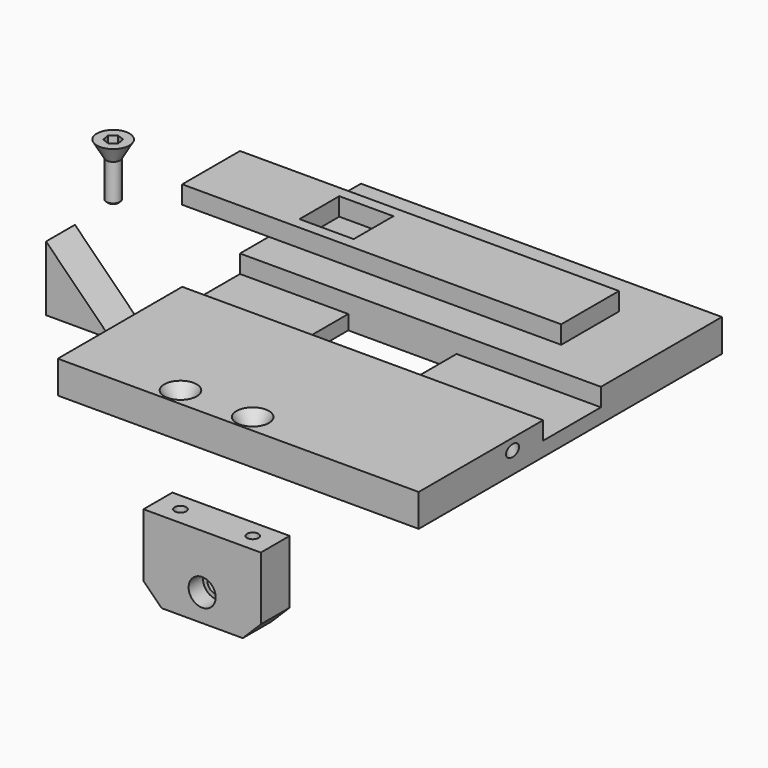
from build123d import *

# Parameters (mm, degrees)
F0_W            = 101.6
F0_H            = 133.35
F1_DEPTH        = 11.43
F3_D            = 4.9149
F3_CSINK_D      = 11.43
F3_CSINK_ANGLE  = 60
F5_W            = 41.275
F5_H            = 12.7
F6_DEPTH        = 28.575
F8_D            = 4.0386
F8_DEPTH        = 9.525
F8_TIP          = 1.213317848
F10_D           = 6.5278
F10_CBORE_D     = 9.525
F10_CBORE_DEPTH = 6.35
F11_W           = 38.1
F11_H           = 25.4
F11_W_2         = 25.4
F12_DEPTH       = 6.35
F13_DEPTH       = 65.406
F15_W           = 101.6
F15_H           = 25.4
F16_DEPTH       = 6.35
F17_W           = 19.05
F17_H           = 17.4752
F18_DEPTH       = 97.156
F20_DEPTH       = 12.7
F21_SIZE2       = 6.34999
F21_SIZE        = 6.34999
F22_DEPTH       = 12.7
F23_DEPTH       = 25.4
F24_DEPTH       = 19.05
F25_SIZE        = 6.35
F28_D           = 4.0386
F28_DEPTH       = 25.4
F28_START       = 31.1992039
F28_TIP         = 1.213317848
F31_SIZE        = 0.508
F33_DEPTH       = 3.175


# Not quite as in the source:
# - a fillet or chamfer is up to 0.001 mm smaller than in the source, because OpenCascade refuses the exact size


with BuildPart() as f1:
    # F0 (on Top) → F1 (new body)
    with BuildSketch(Plane.XY):
        Rectangle(F0_W, F0_H)
    extrude(amount=F1_DEPTH)

    # F3 (through all)
    with Locations(Plane.XY.offset(11.43)):
        with Locations((-12.7, 53.975), (12.7, 53.975), (-12.7, -60.325), (12.7, -60.325)):
            CounterSinkHole(F3_D / 2, F3_CSINK_D / 2, counter_sink_angle=F3_CSINK_ANGLE)

    # F11 (on face) → F12 (cut)
    with BuildSketch(Plane.XY.offset(11.43)):
        with Locations((-31.75, 0.762)):
            Rectangle(F11_W, F11_H)
        with Locations((38.1, 0.762)):
            Rectangle(F11_W_2, F11_H)
    extrude(amount=-F12_DEPTH, mode=Mode.SUBTRACT)

    # F11 (on face) → F13 (cut, through all)
    with BuildSketch(Plane.XY.offset(11.43)):
        with Locations((6.35, 0.762)):
            Rectangle(F11_W, F11_H)
    extrude(amount=-F13_DEPTH, mode=Mode.SUBTRACT)

    # F23 (add): a face of the model
    f23_faces = [f1.faces().sort_by_distance(p)[0] for p in [
        (50.8, 0, 1.338389607),
    ]]
    extrude(f23_faces, amount=F23_DEPTH)

    # F28
    # its depths count from where the whole tool has entered the part; down to there all is cleared
    with Locations(Plane(origin=(71.4375, -71.4375, 0), x_dir=(-0.7071067812, -0.7071067812, 0), z_dir=(0.7071067812, -0.7071067812, 0))):
        with Locations((-35.9150959726, -7.4676)):
            Hole(F28_D / 2, depth=F28_START)
    with Locations(Plane(origin=(71.4375, -71.4375, 0), x_dir=(-0.7071067812, -0.7071067812, 0), z_dir=(0.7071067812, -0.7071067812, 0)).offset(-F28_START)):
        with Locations((-35.9150959726, -7.4676)):
            Hole(F28_D / 2, depth=F28_DEPTH)
            with Locations((0, 0, -(F28_DEPTH + F28_TIP / 2))):  # 118° drill point
                Cone(0, F28_D / 2, F28_TIP, mode=Mode.SUBTRACT)


with BuildPart() as f6:
    # F5 (on offset) → F6 (new body)
    with BuildSketch(Plane(origin=(0, 0, -25.4), x_dir=(1, 0, 0), z_dir=(0, 0, -1))):
        with Locations((0, 60.325)):
            Rectangle(F5_W, F5_H)
    extrude(amount=F6_DEPTH)

    # F8
    with Locations(Plane.XY.offset(-25.4)):
        with Locations((-12.7, -60.325), (12.7, -60.325)):
            Hole(F8_D / 2, depth=F8_DEPTH)
            with Locations((0, 0, -(F8_DEPTH + F8_TIP / 2))):  # 118° drill point
                Cone(0, F8_D / 2, F8_TIP, mode=Mode.SUBTRACT)

    # F10 (through all)
    with Locations(Plane.XZ.offset(66.675)):
        with Locations((0, -44.4415174425)):
            CounterBoreHole(F10_D / 2, F10_CBORE_D / 2, F10_CBORE_DEPTH)

    # F25
    f25_edges = [f6.edges().sort_by_distance(p)[0] for p in [
        (-20.6375, -60.325, -53.975),
        (20.6375, -60.325, -53.975),
    ]]
    chamfer(f25_edges, length=F25_SIZE)


with BuildPart() as f16:
    # F15 (on offset) → F16 (new body)
    with BuildSketch(Plane.XY.offset(36.83)):
        with Locations((0, 0.762)):
            Rectangle(F15_W, F15_H)
    extrude(amount=F16_DEPTH)

    # F17 (on face) → F18 (cut, through all)
    with BuildSketch(Plane.XY.offset(43.18)):
        with Locations((-3.175, 0.762)):
            Rectangle(F17_W, F17_H)
    extrude(amount=-F18_DEPTH, mode=Mode.SUBTRACT)

    # F21 (size 6.35 and 6.35 in the source; OpenCascade refuses exactly that, so slightly less here)
    f21_edges = [f16.edges().sort_by_distance(p)[0] for p in [
        (6.35, 0.762, 36.83),
    ]]
    chamfer(f21_edges, length=F21_SIZE, length2=F21_SIZE2)

    # F22 (add): a face of the model
    f22_faces = [f16.faces().sort_by_distance(p)[0] for p in [
        (50.8, 0.762, 40.005),
    ]]
    extrude(f22_faces, amount=F22_DEPTH)

    # F24 (add): a face of the model
    f24_faces = [f16.faces().sort_by_distance(p)[0] for p in [
        (63.5, 0.762, 40.005),
    ]]
    extrude(f24_faces, amount=F24_DEPTH)


with BuildPart() as f20:
    # F19 (on Front) → F20 (new body)
    with BuildSketch(Plane.XZ):
        Polygon((-75.2351675029, -12.4421706577), (-98.090454936, 10.4131167755), (-98.090454936, -12.4421706577), align=None)
    extrude(amount=F20_DEPTH)


with BuildPart() as f30:
    # F29 (on Front) → F30 (revolve)
    with BuildSketch(Plane.XZ):
        Polygon((-84.6429214931, 41.2107444957), (-90.3579214931, 41.2107444957), (-87.0559214931, 35.4915127291), (-87.0559214931, 22.1607444957), (-84.6429214931, 22.1607444957), align=None)
    revolve(axis=Axis((-84.6429214931, 0, 31.6857444957), (0, 0, -1)))

    # F31
    f31_edges = [f30.edges().sort_by_distance(p)[0] for p in [
        (-82.229921, 0, 22.160744),
    ]]
    chamfer(f31_edges, length=F31_SIZE)

    # F32 (on face) → F33 (cut)
    with BuildSketch(Plane.XY.offset(41.2107444957)):
        Polygon((-84.1775248652, -2.7025184536), (-82.0697735441, -0.9482139242), (-82.535170172, 1.7543045294), (-85.1083181209, 2.7025184536), (-87.216069442, 0.9482139242), (-86.7506728141, -1.7543045294), align=None)
    extrude(amount=-F33_DEPTH, mode=Mode.SUBTRACT)


solid = Compound([f1.part, f6.part, f16.part, f20.part, f30.part])
